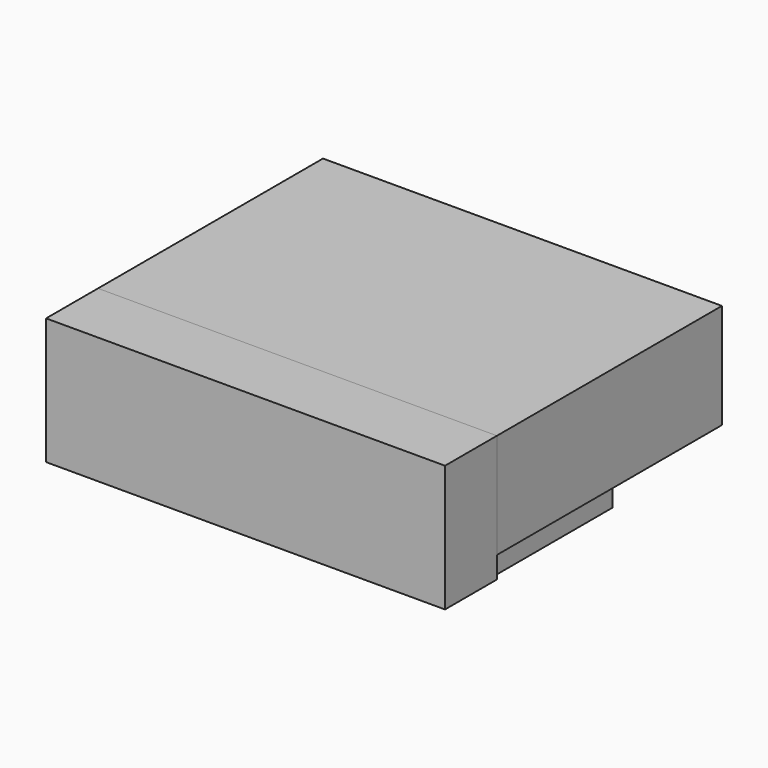
from build123d import *

# Parameters (mm, degrees)
F0_W     = 18.44
F0_H     = 13
F1_DEPTH = 4.85
F2_W     = 1
F2_H     = 7
F3_DEPTH = 1
F4_W     = 18.44
F4_H     = 5.85
F5_DEPTH = 3
F6_W     = 15.94
F6_H     = 1
F7_DEPTH = 7


with BuildPart() as f1:
    # F0 (on Top) → F1 (new body)
    with BuildSketch(Plane.XY):
        with Locations((9.22, 6.5)):
            Rectangle(F0_W, F0_H)
    extrude(amount=F1_DEPTH)

    # F2 (on face) → F3 (join)
    with BuildSketch(Plane(origin=(0, 0, 0), x_dir=(1, 0, 0), z_dir=(0, 0, -1))):
        with Locations((0.75, -3.5)):
            Rectangle(F2_W, F2_H)
        with Locations((17.69, -3.5)):
            Rectangle(F2_W, F2_H)
    extrude(amount=F3_DEPTH)


with BuildPart() as f5:
    # F4 (on face) → F5 (new body)
    with BuildSketch(Plane.XZ):
        with Locations((9.22, 1.925)):
            Rectangle(F4_W, F4_H)
    extrude(amount=F5_DEPTH)

    # F6 (on face) → F7 (join, through all)
    with BuildSketch(Plane(origin=(0, 0, 0), x_dir=(-1, 0, 0), z_dir=(0, 1, 0))):
        with Locations((-9.22, -0.5)):
            Rectangle(F6_W, F6_H)
    extrude(amount=F7_DEPTH)


solid = Compound([f1.part, f5.part])
